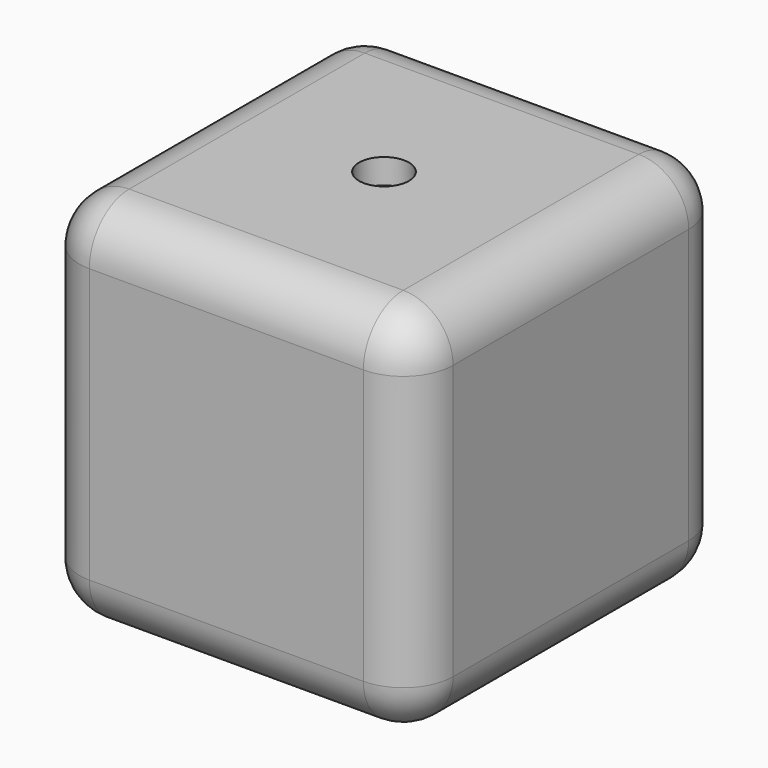
from build123d import *

# Parameters (mm, degrees)
F0_W         = 15
F0_H         = 15.8181820747
F1_DEPTH     = 15
F2_R         = 2
F3_R         = 1
F4_DEPTH     = 1
F5_TEXT_SIZE = 9.498960546
F6_DEPTH     = 0.5


# Not quite as in the source:
# - Text() gives the source's letters only with a copy of the font that has no kerning and outlines rounded to 1/6400 em; it was checked with that copy


with BuildPart() as f1:
    # F0 (on Top) → F1 (new body)
    with BuildSketch(Plane.XY):
        Rectangle(F0_W, F0_H)
    extrude(amount=F1_DEPTH)

    # F2
    f2_edges = [f1.edges().sort_by_distance(p)[0] for p in [
        (0, -7.909091, 15),
        (7.5, 0, 15),
        (0, 7.909091, 15),
        (-7.5, 0, 15),
        (0, -7.909091, 0),
        (7.5, 0, 0),
        (-7.5, -7.909091, 7.5),
        (7.5, -7.909091, 7.5),
        (7.5, 7.909091, 7.5),
        (-7.5, 7.909091, 7.5),
        (-7.5, 0, 0),
        (0, 7.909091, 0),
    ]]
    fillet(f2_edges, radius=F2_R)

    # F3 (on face) → F4 (cut)
    with BuildSketch(Plane.XY.offset(15)):
        Circle(F3_R)
    extrude(amount=-F4_DEPTH, mode=Mode.SUBTRACT)

    # F5 (on face) → F6 (cut)
    with BuildSketch(Plane(origin=(0, 0, 0), x_dir=(1, 0, 0), z_dir=(0, 0, -1))):
        with Locations((-2.8682408211, -3.5)):
            Text('6', F5_TEXT_SIZE, font='Open Sans', font_style=FontStyle.BOLD, text_align=(TextAlign.LEFT, TextAlign.BOTTOM))
    extrude(amount=-F6_DEPTH, mode=Mode.SUBTRACT)


solid = f1.part
